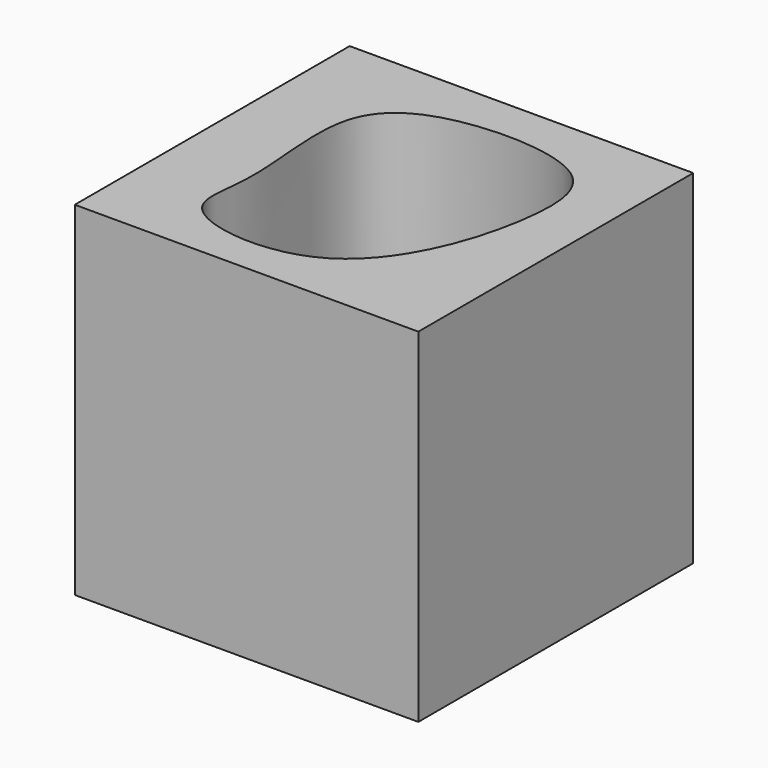
from build123d import *

# Parameters (mm, degrees)
F0_W     = 50.8
F0_H     = 50.8
F1_DEPTH = 50.8


with BuildPart() as f1:
    # F0 (on Top) → F1 (new body)
    with BuildSketch(Plane.XY):
        Rectangle(F0_W, F0_H)
        with BuildLine():
            add(Edge.make_bspline(
                [(14.1806332394, 16.6524872184), (10.0588903346, 19.4105483099), (-4.9050652919, 20.1028182745), (-16.9721686636, 12.5127782489), (-12.4352083107, -7.5708311213), (-16.8369793115, -19.3682649355), (10.2376599564, -22.8016102522), (19.1043867853, 5.3569623238), (17.4162673699, 14.487365131), (14.1806332394, 16.6524872184)],
                knots=[0, 0, 0, 0, 0.1536186479, 0.2775055808, 0.432896605, 0.5422084282, 0.6965612221, 0.8794069034, 1, 1, 1, 1], degree=3))
        make_face(mode=Mode.SUBTRACT)
    extrude(amount=F1_DEPTH)


solid = f1.part
